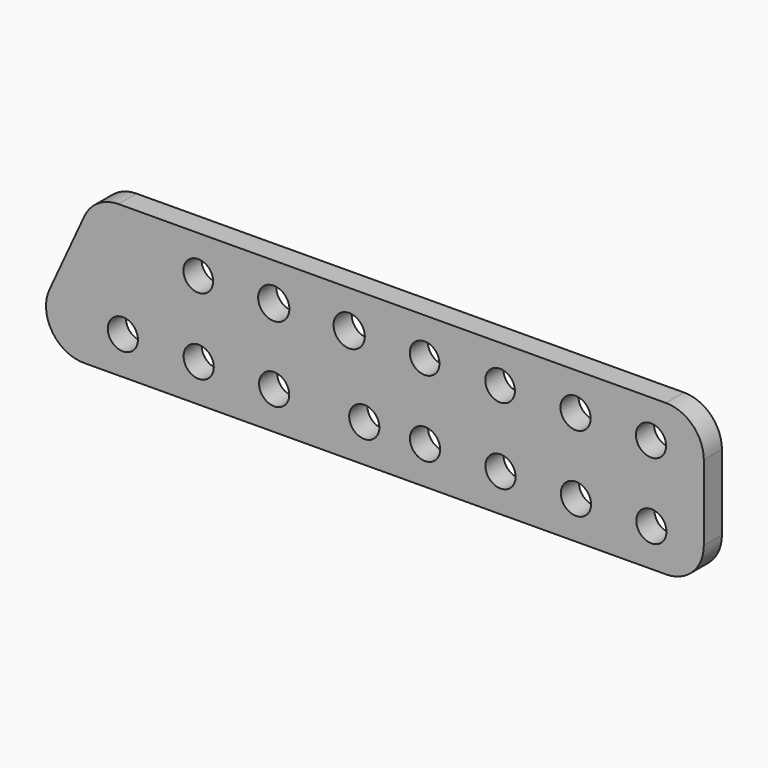
from build123d import *

# Parameters (mm, degrees)
F1_DEPTH = 1.5
F2_R     = 5
F3_R     = 2
F3_R_2   = 1.965178389
F3_R_3   = 2.0701414228
F3_R_4   = 1.9676743652
F4_DEPTH = 25


# Not quite as in the source:
# - a feature names something its author has since deleted; it is built from what else it names


with BuildPart() as f1:
    # F0 (on Front) → F1 (new body, symmetric)
    with BuildSketch(Plane.XZ):
        Polygon((-44.9992595649, -10.2426138069), (45.0007404351, -9.7573861383), (44.9992595649, 10.2426138069), (-35.7811990629, 9.8070925446), align=None)
    extrude(amount=F1_DEPTH, both=True)

    # F2
    f2_edges = [f1.edges().sort_by_distance(p)[0] for p in [
        (45.00074, 0, -9.757386),
        (-35.781199, 0, 9.807093),
        (-44.99926, 0, -10.242614),
        (44.99926, 0, 10.242614),
    ]]
    fillet(f2_edges, radius=F2_R)

    # F3 (on face) → F4 (cut)
    with BuildSketch(Plane.XZ.offset(1.5)):
        with Locations((37.9996325629, 5.2048032201)):
            Circle(F3_R)
        with Locations((27.9996325629, 5.1508890347)):
            Circle(F3_R)
        with Locations((17.9996325629, 5.0969748493)):
            Circle(F3_R_2)
        with Locations((7.9996325629, 5.0430606639)):
            Circle(F3_R_2)
        with Locations((-2.0003674371, 4.9891464785)):
            Circle(F3_R_3)
        with Locations((-12.0003674371, 4.9352322931)):
            Circle(F3_R_3)
        with Locations((-22.0003674371, 4.8813181077)):
            Circle(F3_R_4)
        with Locations((38.0535444404, -4.7947687116)):
            Circle(F3_R)
        with Locations((28.0535444404, -4.848682897)):
            Circle(F3_R)
        with Locations((18.0535444404, -4.9025970824)):
            Circle(F3_R)
        with Locations((8.0535444404, -4.9565112678)):
            Circle(F3_R)
        with Locations((0, -4.9999312966)):
            Circle(F3_R)
        with Locations((-11.9464555596, -5.0643396386)):
            Circle(F3_R)
        with Locations((-21.9464555596, -5.118253824)):
            Circle(F3_R)
        with Locations((-32.0003674371, -5.1724586709)):
            Circle(F3_R)
    extrude(amount=-F4_DEPTH, mode=Mode.SUBTRACT)


solid = f1.part
